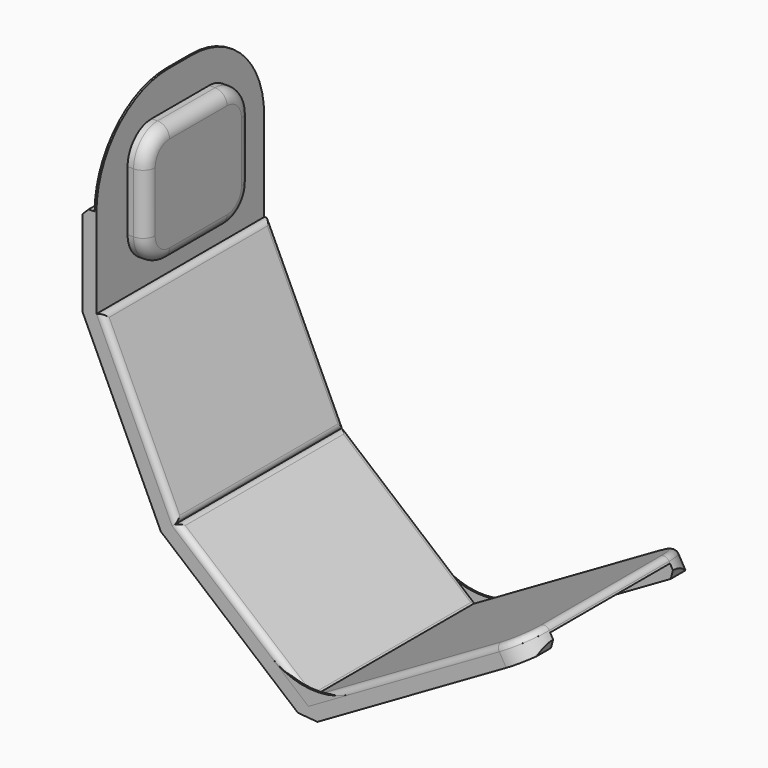
from build123d import *

# Parameters (mm, degrees)
F1_DEPTH     = 175
F2_R         = 150
F4_DEPTH     = 3
F7_DEPTH     = 50
F8_SIZE      = 10
F10_T1_DEPTH = 263
F12_DEPTH    = 30
F13_R        = 20
F14_W        = 350
F14_H        = 298.6698320241
F15_DEPTH    = 10
F16_R        = 9.99999
F17_DEPTH    = 10
F18_R        = 9.99999
F19_DEPTH    = 10
F20_R        = 9.99999
F21_SIZE     = 20


# Not quite as in the source:
# - a fillet or chamfer that OpenCascade refuses, or shapes differently, is made with other operations: its cross-section is extruded or revolved along the edge and cut away or added
# - a fillet or chamfer is up to 0.001 mm smaller than in the source, because OpenCascade refuses the exact size


with BuildPart() as f1:
    # F0 (on Front) → F1 (new body, symmetric)
    with BuildSketch(Plane.XZ):
        Polygon((3, 770), (0, 770), (0, 470), (126.7854785222, 198.107663889), (356.5988114579, 5.271380983), (720.3294810474, 215.271380983), (718.8294810474, 217.8694571944), (356.9180040059, 8.9197685017), (129.2233252444, 199.9782894715), (3, 470.6650839879), align=None)
    extrude(amount=F1_DEPTH, both=True)

    # F2
    f2_edges = [f1.edges().sort_by_distance(p)[0] for p in [
        (1.5, -175, 770),
        (1.5, 175, 770),
    ]]
    fillet(f2_edges, radius=F2_R)

    # F6 (on face) → F7 (join)
    with BuildSketch(Plane.XZ.offset(175)):
        Polygon((0, 470), (0, 620), (-20, 620), (-20, 465.5661067471), (110.5331670407, 185.6368266722), (354.4708611377, -19.0512024747), (730.3294810474, 197.9508729074), (720.3294810474, 215.271380983), (356.5988114579, 5.271380983), (126.7854785222, 198.107663889), align=None)
    extrude(amount=-F7_DEPTH)

    # F8
    f8_edges = [f1.edges().sort_by_distance(p)[0] for p in [
        (-20, -150, 620),
        (730.329481, -150, 197.950873),
    ]]
    chamfer(f8_edges, length=F8_SIZE)

    # F9: F1 across plane


with BuildPart() as f4:
    # F3 (on face) → F4 (new body)
    with BuildSketch(Plane.XZ.offset(175)):
        with BuildLine():
            ThreePointArc((429.6857059273, 50.9322207943), (359.2270167975, 35.3119054774), (292.5511927649, 62.9299360741))
            Line((292.5511927649, 62.9299360741), (356.9180040059, 8.9197685017))
            Line((356.9180040059, 8.9197685017), (429.6857059273, 50.9322207943))
        make_face()
    extrude(amount=-F4_DEPTH)


with BuildPart() as f5_1:
    # F5: instance of F4
    add(f4.part.mirror(Plane.XZ))


with BuildPart() as f1_1:
    add(f1.part)
    add(f1.part.mirror(Plane.XZ))

    # F10: fillet of radius 50 on 2 edges, made by hand

    # F10_s2 → F10_t1 (cut)
    with BuildSketch(Plane(origin=(154.3671279423, 0, -267.3717086146), x_dir=(0, 1, 0), z_dir=(-0.5, 0, 0.8660254038))):
        with BuildLine():
            ThreePointArc((-175, -681.4593201734), (-160.3553390593, -716.8146592327), (-125, -731.4593201734))
            Line((-125, -731.4593201734), (-175, -731.4593201734))
            Line((-175, -731.4593201734), (-175, -681.4593201734))
        make_face()
        with BuildLine():
            ThreePointArc((175, -681.4593201734), (160.3553390593, -716.8146592327), (125, -731.4593201734))
            Line((125, -731.4593201734), (175, -731.4593201734))
            Line((175, -731.4593201734), (175, -681.4593201734))
        make_face()
    extrude(amount=F10_T1_DEPTH, mode=Mode.SUBTRACT)


with BuildPart() as f12:
    # F11 (on face) → F12 (new body)
    with BuildSketch(Plane.YZ.offset(3)):
        with BuildLine():
            Line((-60, 510.6650839879), (60, 510.6650839879))
            ThreePointArc((60, 510.6650839879), (95.3553390593, 525.3097449286), (110, 560.6650839879))
            Line((110, 560.6650839879), (110, 660.6650839879))
            ThreePointArc((110, 660.6650839879), (95.3553390593, 696.0204230473), (60, 710.6650839879))
            Line((60, 710.6650839879), (-60, 710.6650839879))
            ThreePointArc((-60, 710.6650839879), (-95.3553390593, 696.0204230473), (-110, 660.6650839879))
            Line((-110, 660.6650839879), (-110, 560.6650839879))
            ThreePointArc((-110, 560.6650839879), (-95.3553390593, 525.3097449286), (-60, 510.6650839879))
        make_face()
    extrude(amount=F12_DEPTH)

    # F13
    f13_edges = [f12.edges().sort_by_distance(p)[0] for p in [
        (33, -110, 610.665084),
        (33, -95.355339, 525.309745),
        (33, 0, 510.665084),
        (33, 95.355339, 525.309745),
        (33, 110, 610.665084),
        (33, 95.355339, 696.020423),
        (33, 0, 710.665084),
        (33, -95.355339, 696.020423),
    ]]
    fillet(f13_edges, radius=F13_R)


with BuildPart() as f15:
    # F14 (on face) → F15 (new body)
    with BuildSketch(Plane(origin=(182.7393674941, 0, 85.2127665089), x_dir=(0, 1, 0), z_dir=(0.906307787, 0, 0.4226182617))):
        with Locations((0, 275.9646599072)):
            Rectangle(F14_W, F14_H)
    extrude(amount=F15_DEPTH)

    # F16 (radius 10 in the source; OpenCascade refuses exactly that, so slightly less here)
    f16_edges = [f15.edges().sort_by_distance(p)[0] for p in [
        (138.286403, 0, 204.204472),
        (75.17474, 175, 339.547869),
        (12.063078, 0, 474.891267),
        (75.17474, -175, 339.547869),
    ]]
    fillet(f16_edges, radius=F16_R)


with BuildPart() as f17:
    # F17 (new): a face of the model
    f17_faces = [f1_1.part.faces().sort_by_distance(p)[0] for p in [
        (243.0706646252, 0, 104.4490289866),
    ]]
    extrude(f17_faces, amount=F17_DEPTH)

    # F18 (radius 10 in the source; OpenCascade refuses exactly that, so slightly less here)
    f18_edges = [f17.edges().sort_by_distance(p)[0] for p in [
        (249.498541, 175, 112.109473),
        (135.651201, 0, 207.638734),
        (249.498541, -175, 112.109473),
        (363.34588, 0, 16.580213),
    ]]
    fillet(f18_edges, radius=F18_R)


with BuildPart() as f19:
    # F19 (new): a face of the model
    f19_faces = [f1_1.part.faces().sort_by_distance(p)[0] for p in [
        (536.6079070268, 0, 112.6637823815),
    ]]
    extrude(f19_faces, amount=F19_DEPTH)

    # F20 (radius 10 in the source; OpenCascade refuses exactly that, so slightly less here)
    f20_edges = [f19.edges().sort_by_distance(p)[0] for p in [
        (701.146833, 160.355339, 219.207381),
        (713.829481, 0, 226.529711),
        (701.146833, -160.355339, 219.207381),
        (511.223107, -175, 109.554867),
        (351.918004, 0, 17.580023),
        (511.223107, 175, 109.554867),
    ]]
    fillet(f20_edges, radius=F20_R)


with BuildPart() as f1_2:
    add(f1_1.part)

    # F21
    f21_edges = [f1_2.edges().sort_by_distance(p)[0] for p in [
        (354.470861, -150, -19.051202),
        (354.470861, 150, -19.051202),
    ]]
    chamfer(f21_edges, length=F21_SIZE)


solid = Compound([f4.part, f5_1.part, f12.part, f15.part, f17.part, f19.part, f1_2.part])
